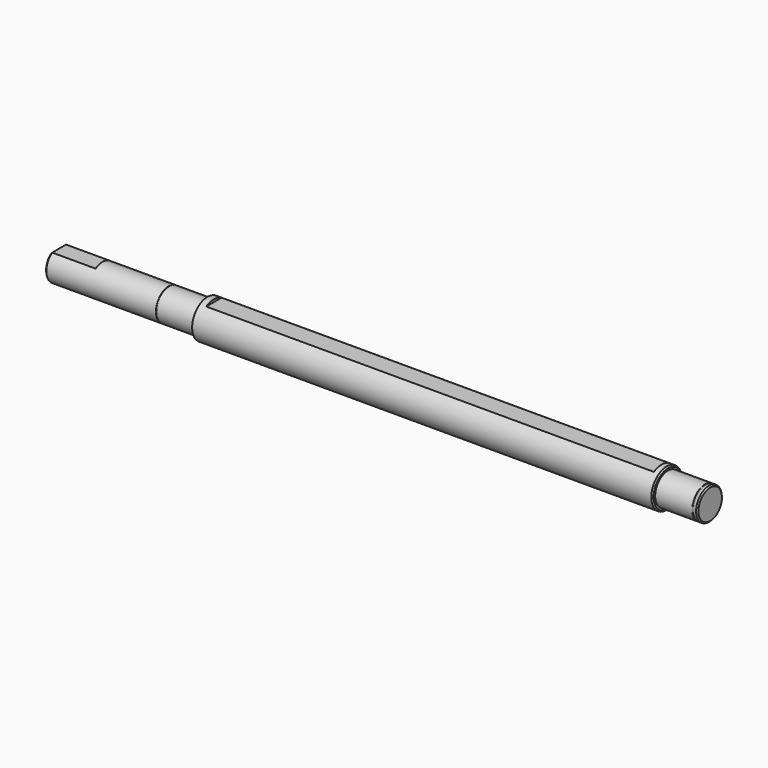
from build123d import *

# Parameters (mm, degrees)
F0_W     = 0.3
F0_H     = 11.95
F0_W_2   = 1.3
F4_DEPTH = 350
F6_DEPTH = 35
F7_SIZE2 = 1
F7_SIZE  = 1


with BuildPart() as f1:
    # F0 (on Front) → F1 (revolve)
    with BuildSketch(Plane.XZ):
        Polygon((-30, 0), (0, 0), (0, 12.5), (-30, 12.5), (-30, 12.225), (-30, 0.275), align=None)
        Polygon((0, 12.5), (0, 0), (360, 0), (360, 12.5), (360, 15), (0, 15), align=None)
        Polygon((360, 12.5), (360, 0), (389, 0), (389, 0.275), (389, 12.225), (389, 12.5), align=None)
        with Locations((-30.15, 6.25)):
            Rectangle(F0_W, F0_H)
        Polygon((-30.3, 0), (-30.3, 0.275), (-30.3, 12.225), (-30.3, 12.5), (-117, 12.5), (-117, 0), align=None)
        with Locations((389.65, 6.25)):
            Rectangle(F0_W_2, F0_H)
        Polygon((390.3, 12.225), (390.3, 0.275), (390.3, 0), (393, 0), (393, 12.5), (390.3, 12.5), align=None)
    revolve(axis=Axis((165, 0, 0), (1, 0, 0)))

    # F3 (on offset) → F4 (cut)
    with BuildSketch(Plane.YZ.offset(355)):
        with BuildLine():
            ThreePointArc((7.4833147735, 13), (0, 15), (-7.4833147735, 13))
            Line((-7.4833147735, 13), (7.4833147735, 13))
        make_face()
        with BuildLine():
            Line((7.4833147735, -13), (-7.4833147735, -13))
            ThreePointArc((-7.4833147735, -13), (0, -15), (7.4833147735, -13))
        make_face()
    extrude(amount=-F4_DEPTH, mode=Mode.SUBTRACT)

    # F5 (on face) → F6 (cut)
    with BuildSketch(Plane(origin=(-117, 0, 0), x_dir=(0, -1, 0), z_dir=(-1, 0, 0))):
        with BuildLine():
            ThreePointArc((6.7823299831, 10.5), (0, 12.5), (-6.7823299831, 10.5))
            Line((-6.7823299831, 10.5), (6.7823299831, 10.5))
        make_face()
        with BuildLine():
            Line((6.7823299831, -10.5), (-6.7823299831, -10.5))
            ThreePointArc((-6.7823299831, -10.5), (0, -12.5), (6.7823299831, -10.5))
        make_face()
    extrude(amount=-F6_DEPTH, mode=Mode.SUBTRACT)

    # F7
    f7_edges = [f1.edges().sort_by_distance(p)[0] for p in [
        (-117, 0, 10.5),
        (-117, 12.5, 0),
        (-117, 0, -10.5),
        (-117, -12.5, 0),
        (393, 0, -12.5),
        (360, 0, -15),
    ]]
    chamfer(f7_edges, length=F7_SIZE, length2=F7_SIZE2)


solid = f1.part
